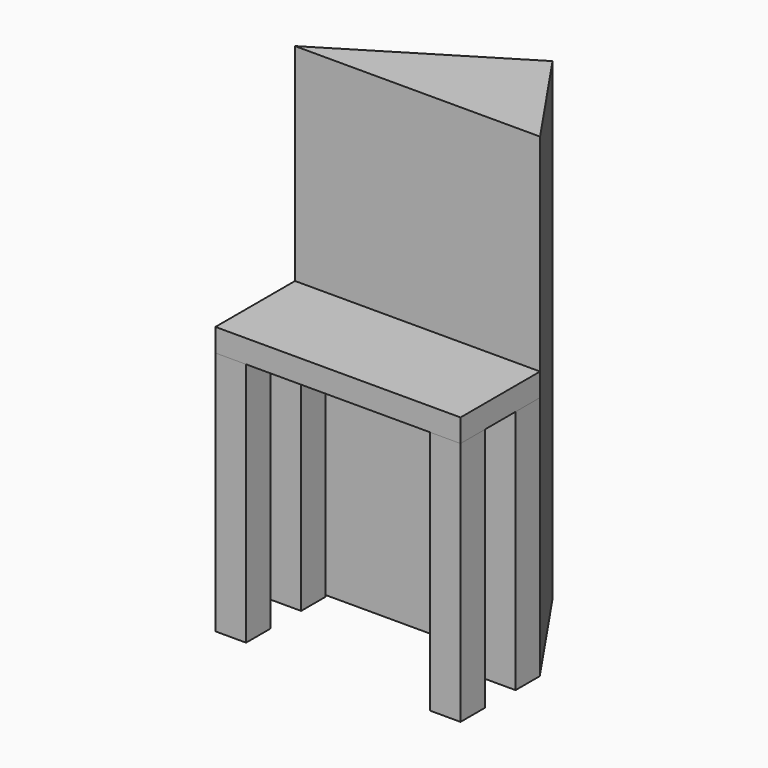
from build123d import *

# Parameters (mm, degrees)
F0_W          = 50.8
F0_H          = 50.8
F1_DEPTH      = 406.4
F2_W          = 203.2
F2_H          = 82.4469551444
F2_W_2        = 50.8
F2_H_2        = 50.8
F7_DEPTH      = 38.1
F9_DEPTH      = 342.9
F9_DEPTH_BACK = 441.96


# Not quite as in the source:
# - a feature names something its author has since deleted; it is built from what else it names


with BuildPart() as f1:
    # F0 (on Top) → F1 (new body)
    with BuildSketch(Plane.XY):
        with Locations((25.4, 25.4)):
            Rectangle(F0_W, F0_H)
    extrude(amount=F1_DEPTH)


with BuildPart() as f5_1:
    # F5: instance of F1
    add(f1.part.mirror(Plane.XZ.offset(-82.4469551444)))


with BuildPart() as f6_1:
    # F6: instance of F5_1
    add(f5_1.part.mirror(Plane.YZ.offset(203.2)))


with BuildPart() as f6_2:
    # F6: instance of F1
    add(f1.part.mirror(Plane.YZ.offset(203.2)))


with BuildPart() as f7:
    # F2 (on face) → F7 (new body)
    with BuildSketch(Plane.XY.offset(406.4)):
        with Locations((304.8, 41.2234775722)):
            Rectangle(F2_W, F2_H)
        with Locations((101.6, 123.6704327166)):
            Rectangle(F2_W, F2_H)
        Polygon((50.8, 50.8), (50.8, 0), (203.2, 0), (203.2, 82.4469551444), (0, 82.4469551444), (0, 50.8), align=None)
        with Locations((304.8, 123.6704327166)):
            Rectangle(F2_W, F2_H)
        with Locations((25.4, 25.4)):
            Rectangle(F2_W_2, F2_H_2)
    extrude(amount=F7_DEPTH)

    # F8 (on face) → F9 (join, two sides)
    with BuildSketch(Plane.XY.offset(444.5)) as f9_sk:
        Polygon((286.7561876774, 340.3366804123), (0, 164.8939102888), (406.4, 164.8939102888), align=None)
    extrude(amount=F9_DEPTH)
    extrude(f9_sk.sketch, amount=-F9_DEPTH_BACK)


solid = Compound([f1.part, f5_1.part, f6_1.part, f6_2.part, f7.part])
